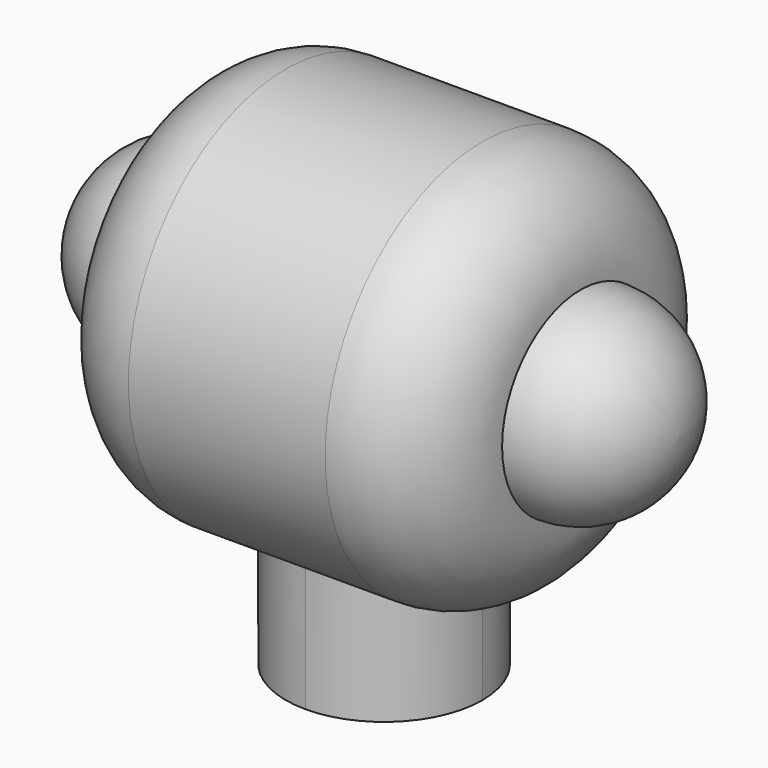
from build123d import *

# Parameters (mm, degrees)
F1_DEPTH      = 15
F1_DEPTH_BACK = 15
F2_DEPTH      = 10
F2_DEPTH_BACK = 10
F3_DEPTH      = 5
F3_DEPTH_BACK = 5
F4_R          = 4.99999
F5_T8_DEPTH   = 31.3397459622
F5_S9_R       = 10
F5_T10_DEPTH  = 18
F5_T14_DEPTH  = 31.3397459622
F5_S15_R      = 10
F5_T16_DEPTH  = 18
F5_T20_DEPTH  = 31.3397459622
F5_S21_R      = 10
F5_T22_DEPTH  = 18
F5_T26_DEPTH  = 31.3397459622
F5_S27_R      = 10
F5_T28_DEPTH  = 18


# Not quite as in the source:
# - a fillet or chamfer that OpenCascade refuses, or shapes differently, is made with other operations: its cross-section is extruded or revolved along the edge and cut away or added
# - a fillet or chamfer is up to 0.001 mm smaller than in the source, because OpenCascade refuses the exact size


with BuildPart() as f1:
    # F0 (on Right) → F1 (new body, two sides)
    with BuildSketch(Plane.YZ) as f1_sk:
        with BuildLine():
            Line((-5, 16.4746102661), (5, 16.4746102661))
            ThreePointArc((5, 16.4746102661), (0, 21.4746102661), (-5, 16.4746102661))
        make_face()
        with BuildLine():
            ThreePointArc((-5, 16.4746102661), (0, 11.4746102661), (5, 16.4746102661))
            Line((5, 16.4746102661), (-5, 16.4746102661))
        make_face()
    extrude(amount=F1_DEPTH)
    extrude(f1_sk.sketch, amount=-F1_DEPTH_BACK)

    # F0 (on Right) → F2 (join, two sides)
    with BuildSketch(Plane.YZ) as f2_sk:
        with BuildLine():
            ThreePointArc((-5, 16.4746102661), (0, 21.4746102661), (5, 16.4746102661))
            Line((5, 16.4746102661), (5, 7.8143562283))
            ThreePointArc((5, 7.8143562283), (8.6602540378, 11.4746102661), (10, 16.4746102661))
            ThreePointArc((10, 16.4746102661), (-5, 25.1348643039), (-5, 7.8143562283))
            Line((-5, 7.8143562283), (-5, 16.4746102661))
        make_face()
        with BuildLine():
            Line((5, 7.8143562283), (5, 16.4746102661))
            ThreePointArc((5, 16.4746102661), (0, 11.4746102661), (-5, 16.4746102661))
            Line((-5, 16.4746102661), (-5, 7.8143562283))
            ThreePointArc((-5, 7.8143562283), (0, 6.4746102661), (5, 7.8143562283))
        make_face()
    extrude(amount=F2_DEPTH)
    extrude(f2_sk.sketch, amount=-F2_DEPTH_BACK)

    # F0 (on Right) → F3 (join, two sides)
    with BuildSketch(Plane.YZ) as f3_sk:
        with BuildLine():
            Line((5, 1.4746102661), (5, 7.8143562283))
            ThreePointArc((5, 7.8143562283), (0, 6.4746102661), (-5, 7.8143562283))
            Line((-5, 7.8143562283), (-5, 1.4746102661))
            Line((-5, 1.4746102661), (5, 1.4746102661))
        make_face()
    extrude(amount=F3_DEPTH)
    extrude(f3_sk.sketch, amount=-F3_DEPTH_BACK)

    # F4 (radius 5 in the source; OpenCascade refuses exactly that, so slightly less here)
    f4_edges = [f1.edges().sort_by_distance(p)[0] for p in [
        (15, 5, 16.47461),
        (-15, 5, 16.47461),
    ]]
    fillet(f4_edges, radius=F4_R)

    # F5: fillet of radius 5 on 8 edges, made by hand

    # F5_s1 → F5_t2 (revolve, cut)
    with BuildSketch(Plane.XY.offset(16.4746102661)):
        with BuildLine():
            ThreePointArc((-5, 10), (-8.5355339059, 8.5355339059), (-10, 5))
            Line((-10, 5), (-10, 10))
            Line((-10, 10), (-5, 10))
        make_face()
    revolve(axis=Axis((-10, 0, 16.4746102661), (1, 0, 0)), mode=Mode.SUBTRACT)

    # F5_s3 → F5_t4 (revolve, cut)
    with BuildSketch(Plane.XY.offset(16.4746102661)):
        with BuildLine():
            ThreePointArc((10, 5), (8.5355339059, 8.5355339059), (5, 10))
            Line((5, 10), (10, 10))
            Line((10, 10), (10, 5))
        make_face()
    revolve(axis=Axis((10, 0, 16.4746102661), (1, 0, 0)), mode=Mode.SUBTRACT)


with BuildPart() as f5_tool6:
    # F5_s7 → F5_t8 (new body)
    with BuildSketch(Plane.XY.offset(-11.0253897339)):
        with BuildLine():
            ThreePointArc((-5, 0), (-3.5355339059, 3.5355339059), (0, 5))
            Line((0, 5), (-5, 5))
            Line((-5, 5), (-5, 0))
        make_face()
    extrude(amount=F5_T8_DEPTH)

    # F5_s9 → F5_t10 (cut, symmetric)
    with BuildSketch(Plane.YZ.offset(-2.5)):
        with Locations((0, 16.4746102661)):
            Circle(F5_S9_R)
    extrude(amount=F5_T10_DEPTH, both=True, mode=Mode.SUBTRACT)


with BuildPart() as f1_1:
    add(f1.part)

    # F5_t5: cut F5_tool6
    add(f5_tool6.part, mode=Mode.SUBTRACT)


with BuildPart() as f5_tool12:
    # F5_s13 → F5_t14 (new body)
    with BuildSketch(Plane.XY.offset(-11.0253897339)):
        with BuildLine():
            ThreePointArc((0, 5), (3.5355339059, 3.5355339059), (5, 0))
            Line((5, 0), (5, 5))
            Line((5, 5), (0, 5))
        make_face()
    extrude(amount=F5_T14_DEPTH)

    # F5_s15 → F5_t16 (cut, symmetric)
    with BuildSketch(Plane.YZ.offset(2.5)):
        with Locations((0, 16.4746102661)):
            Circle(F5_S15_R)
    extrude(amount=F5_T16_DEPTH, both=True, mode=Mode.SUBTRACT)


with BuildPart() as f1_2:
    add(f1_1.part)

    # F5_t11: cut F5_tool12
    add(f5_tool12.part, mode=Mode.SUBTRACT)


with BuildPart() as f5_tool18:
    # F5_s19 → F5_t20 (new body)
    with BuildSketch(Plane.XY.offset(20.3143562283)):
        with BuildLine():
            ThreePointArc((0, -5), (3.5355339059, -3.5355339059), (5, 0))
            Line((5, 0), (5, -5))
            Line((5, -5), (0, -5))
        make_face()
    extrude(amount=-F5_T20_DEPTH)

    # F5_s21 → F5_t22 (cut, symmetric)
    with BuildSketch(Plane.YZ.offset(2.5)):
        with Locations((0, 16.4746102661)):
            Circle(F5_S21_R)
    extrude(amount=F5_T22_DEPTH, both=True, mode=Mode.SUBTRACT)


with BuildPart() as f1_3:
    add(f1_2.part)

    # F5_t17: cut F5_tool18
    add(f5_tool18.part, mode=Mode.SUBTRACT)


with BuildPart() as f5_tool24:
    # F5_s25 → F5_t26 (new body)
    with BuildSketch(Plane.XY.offset(20.3143562283)):
        with BuildLine():
            ThreePointArc((0, -5), (-3.5355339059, -3.5355339059), (-5, 0))
            Line((-5, 0), (-5, -5))
            Line((-5, -5), (0, -5))
        make_face()
    extrude(amount=-F5_T26_DEPTH)

    # F5_s27 → F5_t28 (cut, symmetric)
    with BuildSketch(Plane.YZ.offset(-2.5)):
        with Locations((0, 16.4746102661)):
            Circle(F5_S27_R)
    extrude(amount=F5_T28_DEPTH, both=True, mode=Mode.SUBTRACT)


with BuildPart() as f1_4:
    add(f1_3.part)

    # F5_t23: cut F5_tool24
    add(f5_tool24.part, mode=Mode.SUBTRACT)


solid = f1_4.part
